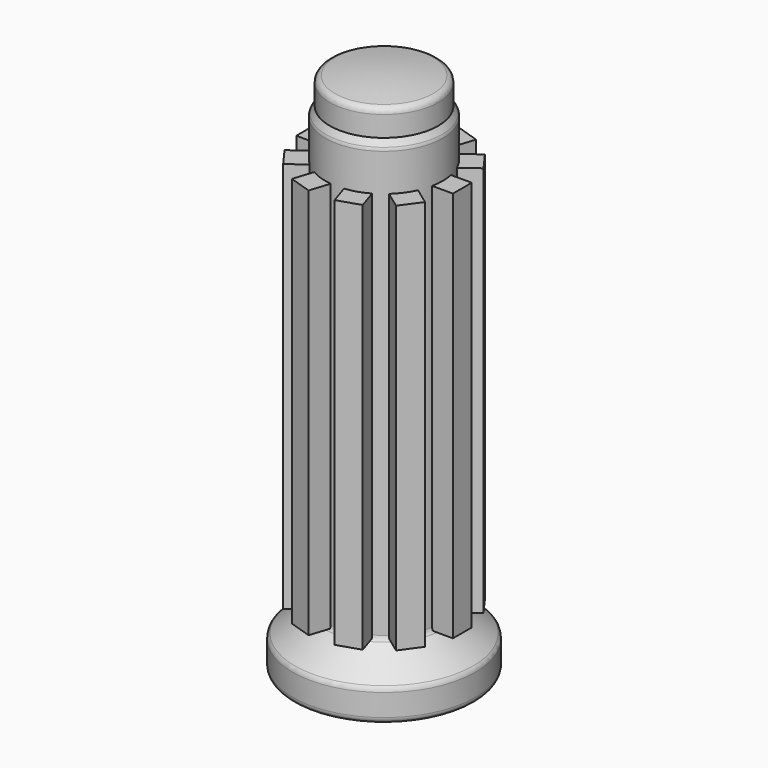
from build123d import *

# Parameters (mm, degrees)
F2_R          = 1.6
F5_END_RADIUS = 15
F4_W          = 6
F4_H          = 100
F5_REACH      = 143.5231135391
F6_COUNT      = 10


with BuildPart() as f1:
    # F0 (on Front) → F1 (revolve)
    with BuildSketch(Plane.XZ):
        with BuildLine():
            ThreePointArc((13.8452994616, 133.5755787269), (6.9591898441, 134.6429573327), (0, 135))
            Line((0, 135), (0, 125))
            Line((0, 125), (10.75, 125))
            Line((10.75, 125), (10.75, 0))
            Line((10.75, 0), (23.3422751482, 0))
            Line((23.3422751482, 0), (23.3422751482, 8))
            Line((23.3422751482, 8), (15, 15))
            Line((15, 15), (15, 125))
            Line((15, 125), (13.8452994616, 127))
            Line((13.8452994616, 127), (13.8452994616, 133.5755787269))
        make_face()
    revolve(axis=Axis((0, 0, 2.9858769252), (0, 0, -1)))

    # F2
    f2_edges = [f1.edges().sort_by_distance(p)[0] for p in [
        (-13.845299, 0, 133.575579),
        (-15, 0, 125),
        (-23.342275, 0, 8),
        (-23.342275, 0, 0),
        (-15, 0, 15),
    ]]
    fillet(f2_edges, radius=F2_R)


with BuildPart() as f5:
    f5_end = (Plane.XY.offset(70.1586867727) * Cylinder(F5_END_RADIUS, 587.6050042205, mode=Mode.PRIVATE)).faces().sort_by_distance((-15, 0, 70.1586867727))[0]
    # F4 (on offset) → F5 (new body, up to the whole of a round face its end follows)
    with BuildSketch(Plane.YZ.offset(20)):
        with Locations((0, 65)):
            Rectangle(F4_W, F4_H)
    f5_long = extrude(amount=-F5_REACH, mode=Mode.PRIVATE)
    add(split(f5_long, bisect_by=f5_end, keep=Keep.ALL, mode=Mode.PRIVATE).solids().sort_by_distance((20, 0, 65))[0])


with BuildPart() as f6_1:
    # F6: instance of F5
    add(f5.part.rotate(Axis((0, 0, 15), (0, 0, 1)), 1 * 360 / F6_COUNT))


with BuildPart() as f6_2:
    # F6: instance of F5
    add(f5.part.rotate(Axis((0, 0, 15), (0, 0, 1)), 2 * 360 / F6_COUNT))


with BuildPart() as f6_3:
    # F6: instance of F5
    add(f5.part.rotate(Axis((0, 0, 15), (0, 0, 1)), 3 * 360 / F6_COUNT))


with BuildPart() as f6_4:
    # F6: instance of F5
    add(f5.part.rotate(Axis((0, 0, 15), (0, 0, 1)), 4 * 360 / F6_COUNT))


with BuildPart() as f6_5:
    # F6: instance of F5
    add(f5.part.rotate(Axis((0, 0, 15), (0, 0, 1)), 5 * 360 / F6_COUNT))


with BuildPart() as f6_6:
    # F6: instance of F5
    add(f5.part.rotate(Axis((0, 0, 15), (0, 0, 1)), 6 * 360 / F6_COUNT))


with BuildPart() as f6_7:
    # F6: instance of F5
    add(f5.part.rotate(Axis((0, 0, 15), (0, 0, 1)), 7 * 360 / F6_COUNT))


with BuildPart() as f6_8:
    # F6: instance of F5
    add(f5.part.rotate(Axis((0, 0, 15), (0, 0, 1)), 8 * 360 / F6_COUNT))


with BuildPart() as f6_9:
    # F6: instance of F5
    add(f5.part.rotate(Axis((0, 0, 15), (0, 0, 1)), 9 * 360 / F6_COUNT))


solid = Compound([f1.part, f5.part, f6_1.part, f6_2.part, f6_3.part, f6_4.part, f6_5.part, f6_6.part, f6_7.part, f6_8.part, f6_9.part])
